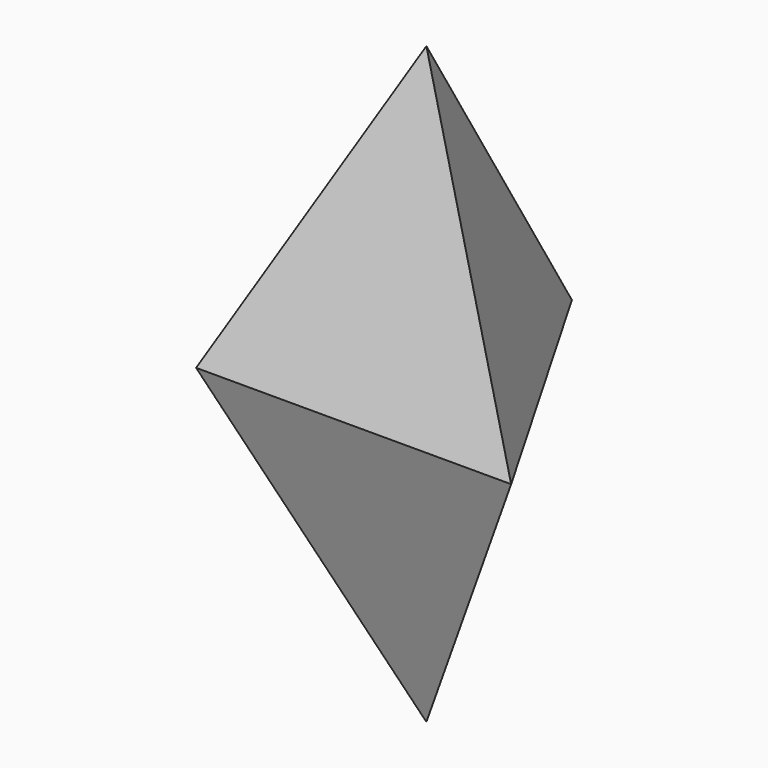
from build123d import *


# Not quite as in the source:
# - an extrude whose draft closes it to a point is written as a loft to that point


with BuildPart() as f1:
    # F0 (on Top) → F1 section 0
    with BuildSketch(Plane.XY, mode=Mode.PRIVATE) as f1_s0:
        Polygon((0, 21.9970452561), (-12.7, 0), (12.7, 0), align=None)
    loft([f1_s0.sketch, Vertex(0, 7.3323484187, 23.983031025)], ruled=True)

    # F1_face (on face) → F2 section 0
    with BuildSketch(Plane(origin=(0, 7.3323484187, 0), x_dir=(1, 0, 0), z_dir=(0, 0, -1)), mode=Mode.PRIVATE) as f2_s0:
        Polygon((-12.7, 7.3323484187), (0, -14.6646968374), (12.7, 7.3323484187), align=None)
    loft([f2_s0.sketch, Vertex(0, 7.3323484187, -23.983031025)], ruled=True)


solid = f1.part
